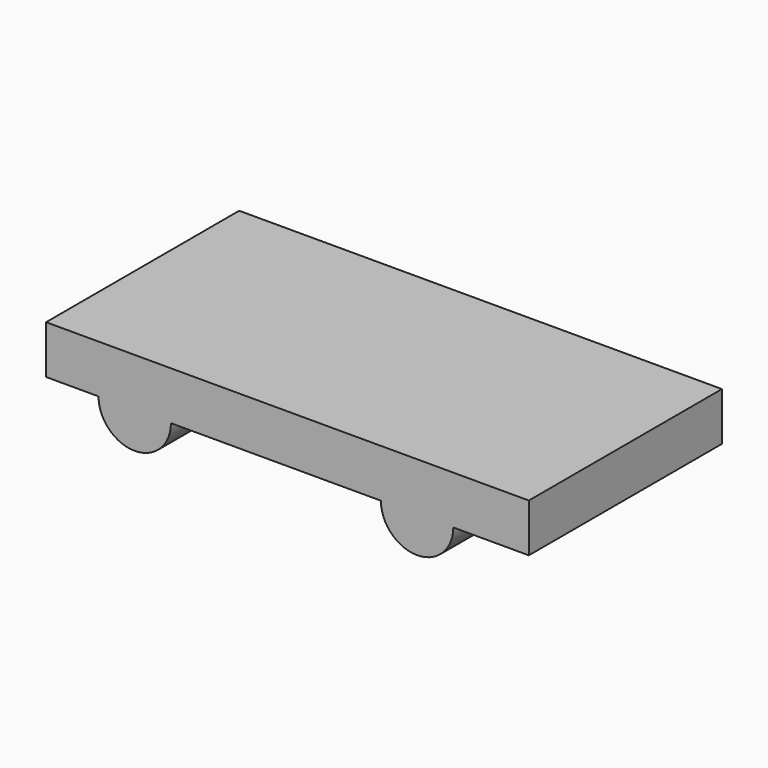
from build123d import *

# Parameters (mm, degrees)
F0_W     = 127
F0_H     = 63.5
F1_DEPTH = 12.7
F4_DEPTH = 63.5


with BuildPart() as f1:
    # F0 (on Top) → F1 (new body)
    with BuildSketch(Plane.XY):
        Rectangle(F0_W, F0_H)
    extrude(amount=F1_DEPTH)

    # F2 (on face) + F3 (on face) → F4 (join)
    with BuildSketch(Plane.XZ.offset(31.75)):
        with BuildLine():
            ThreePointArc((-49.7021888137, 0), (-40.1771888137, -9.525), (-30.6521888137, 0))
            Line((-30.6521888137, 0), (-49.7021888137, 0))
        make_face()
    with BuildSketch(Plane.XZ.offset(31.75)):
        with BuildLine():
            Line((24.5841778814, 0), (43.6341778814, 0))
            ThreePointArc((43.6341778814, 0), (34.1091778814, 9.525), (24.5841778814, 0))
        make_face()
        with BuildLine():
            ThreePointArc((24.5841778814, 0), (34.1091778814, -9.525), (43.6341778814, 0))
            Line((43.6341778814, 0), (24.5841778814, 0))
        make_face()
    extrude(amount=-F4_DEPTH)


solid = f1.part
